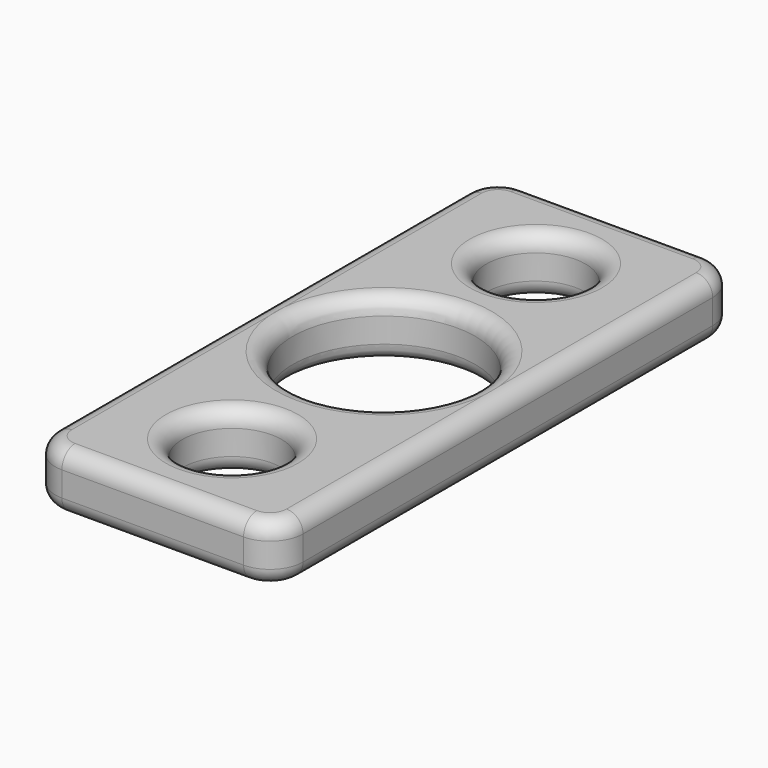
from build123d import *

# Parameters (mm, degrees)
F0_W         = 30
F0_H         = 70
F0_R         = 5.9998479486
F0_R_2       = 11.05
F1_DEPTH     = 7
F2_T1_DEPTH  = 80
F2_T3_DEPTH  = 40
F3_T1_DEPTH  = 6.9999999998
F3_T4_ANGLE  = 90
F3_T6_ANGLE  = 90
F3_T8_ANGLE  = 90
F3_T10_ANGLE = 90
F3_T12_ANGLE = 90
F3_T14_ANGLE = 90
F3_T16_ANGLE = 90
F3_T18_ANGLE = 90


# Not quite as in the source:
# - a fillet or chamfer that OpenCascade refuses, or shapes differently, is made with other operations: its cross-section is extruded or revolved along the edge and cut away or added


with BuildPart() as f1:
    # F0 (on Top) → F1 (new body)
    with BuildSketch(Plane.XY):
        Rectangle(F0_W, F0_H)
        with Locations((0, -23)):
            Circle(F0_R, mode=Mode.SUBTRACT)
        Circle(F0_R_2, mode=Mode.SUBTRACT)
        with Locations((0, 23)):
            Circle(F0_R, mode=Mode.SUBTRACT)
    extrude(amount=F1_DEPTH)

    # F2: fillet of radius 2 on 14 edges, made by hand

    # F2_s2 → F2_t1 (cut)
    with BuildSketch(Plane.XZ.offset(-40)):
        with BuildLine():
            ThreePointArc((15, 5), (14.4142135624, 6.4142135624), (13, 7))
            Line((13, 7), (15, 7))
            Line((15, 7), (15, 5))
        make_face()
        with BuildLine():
            ThreePointArc((-15, 5), (-14.4142135624, 6.4142135624), (-13, 7))
            Line((-13, 7), (-15, 7))
            Line((-15, 7), (-15, 5))
        make_face()
        with BuildLine():
            ThreePointArc((15, 2), (14.4142135624, 0.5857864376), (13, 0))
            Line((13, 0), (15, 0))
            Line((15, 0), (15, 2))
        make_face()
        with BuildLine():
            ThreePointArc((-15, 2), (-14.4142135624, 0.5857864376), (-13, 0))
            Line((-13, 0), (-15, 0))
            Line((-15, 0), (-15, 2))
        make_face()
    extrude(amount=F2_T1_DEPTH, mode=Mode.SUBTRACT)

    # F2_s4 → F2_t3 (cut)
    with BuildSketch(Plane.YZ.offset(-20)):
        with BuildLine():
            ThreePointArc((35, 5), (34.4142135624, 6.4142135624), (33, 7))
            Line((33, 7), (35, 7))
            Line((35, 7), (35, 5))
        make_face()
        with BuildLine():
            ThreePointArc((-35, 5), (-34.4142135624, 6.4142135624), (-33, 7))
            Line((-33, 7), (-35, 7))
            Line((-35, 7), (-35, 5))
        make_face()
        with BuildLine():
            ThreePointArc((35, 2), (34.4142135624, 0.5857864376), (33, 0))
            Line((33, 0), (35, 0))
            Line((35, 0), (35, 2))
        make_face()
        with BuildLine():
            ThreePointArc((-35, 2), (-34.4142135624, 0.5857864376), (-33, 0))
            Line((-33, 0), (-35, 0))
            Line((-35, 0), (-35, 2))
        make_face()
    extrude(amount=F2_T3_DEPTH, mode=Mode.SUBTRACT)

    # F2_s5 → F2_t6 (revolve, cut)
    with BuildSketch(Plane.XZ.offset(23)):
        with BuildLine():
            ThreePointArc((5.9998479486, 5), (6.5856343863, 6.4142135624), (7.9998479486, 7))
            Line((7.9998479486, 7), (5.9998479486, 7))
            Line((5.9998479486, 7), (5.9998479486, 5))
        make_face()
    revolve(axis=Axis((0, -23, 7), (0, 0, 1)), mode=Mode.SUBTRACT)

    # F2_s7 → F2_t8 (revolve, cut)
    with BuildSketch(Plane.XZ):
        with BuildLine():
            ThreePointArc((11.05, 5), (11.6357864376, 6.4142135624), (13.05, 7))
            Line((13.05, 7), (11.05, 7))
            Line((11.05, 7), (11.05, 5))
        make_face()
    revolve(axis=Axis((0, 0, 7), (0, 0, 1)), mode=Mode.SUBTRACT)

    # F2_s9 → F2_t10 (revolve, cut)
    with BuildSketch(Plane.XZ.offset(-23)):
        with BuildLine():
            ThreePointArc((5.9998479486, 5), (6.5856343863, 6.4142135624), (7.9998479486, 7))
            Line((7.9998479486, 7), (5.9998479486, 7))
            Line((5.9998479486, 7), (5.9998479486, 5))
        make_face()
    revolve(axis=Axis((0, 23, 7), (0, 0, 1)), mode=Mode.SUBTRACT)

    # F2_s11 → F2_t12 (revolve, cut)
    with BuildSketch(Plane.XZ.offset(23)):
        with BuildLine():
            ThreePointArc((5.9998479486, 2), (6.5856343863, 0.5857864376), (7.9998479486, 0))
            Line((7.9998479486, 0), (5.9998479486, 0))
            Line((5.9998479486, 0), (5.9998479486, 2))
        make_face()
    revolve(axis=Axis((0, -23, 0), (0, 0, 1)), mode=Mode.SUBTRACT)

    # F2_s13 → F2_t14 (revolve, cut)
    with BuildSketch(Plane.XZ):
        with BuildLine():
            ThreePointArc((11.05, 2), (11.6357864376, 0.5857864376), (13.05, 0))
            Line((13.05, 0), (11.05, 0))
            Line((11.05, 0), (11.05, 2))
        make_face()
    revolve(axis=Axis((0, 0, 0), (0, 0, 1)), mode=Mode.SUBTRACT)

    # F2_s15 → F2_t16 (revolve, cut)
    with BuildSketch(Plane.XZ.offset(-23)):
        with BuildLine():
            ThreePointArc((5.9998479486, 2), (6.5856343863, 0.5857864376), (7.9998479486, 0))
            Line((7.9998479486, 0), (5.9998479486, 0))
            Line((5.9998479486, 0), (5.9998479486, 2))
        make_face()
    revolve(axis=Axis((0, 23, 0), (0, 0, 1)), mode=Mode.SUBTRACT)

    # F3: fillet of radius 4 on 4 edges, made by hand

    # F3_s2 → F3_t1 (cut)
    with BuildSketch(Plane.XY):
        with BuildLine():
            ThreePointArc((-11, -35), (-13.8284271247, -33.8284271247), (-15, -31))
            Line((-15, -31), (-15, -35))
            Line((-15, -35), (-11, -35))
        make_face()
        with BuildLine():
            ThreePointArc((15, -31), (13.8284271247, -33.8284271247), (11, -35))
            Line((11, -35), (15, -35))
            Line((15, -35), (15, -31))
        make_face()
        with BuildLine():
            ThreePointArc((15, 31), (13.8284271247, 33.8284271247), (11, 35))
            Line((11, 35), (15, 35))
            Line((15, 35), (15, 31))
        make_face()
        with BuildLine():
            ThreePointArc((-11, 35), (-13.8284271247, 33.8284271247), (-15, 31))
            Line((-15, 31), (-15, 35))
            Line((-15, 35), (-11, 35))
        make_face()
    extrude(amount=F3_T1_DEPTH, mode=Mode.SUBTRACT)

    # F3_s3 → F3_t4 (revolve, cut)
    with BuildSketch(Plane.XZ.offset(-31)):
        with BuildLine():
            ThreePointArc((-13.0000000001, 0), (-14.4142135624, 0.5857864376), (-15, 1.9999999999))
            Line((-15, 1.9999999999), (-15, 0))
            Line((-15, 0), (-13.0000000001, 0))
        make_face()
    revolve(axis=Axis((-11, 31, 0), (0, 0, -1)), revolution_arc=F3_T4_ANGLE, mode=Mode.SUBTRACT)

    # F3_s5 → F3_t6 (revolve, cut)
    with BuildSketch(Plane.YZ.offset(-11)):
        with BuildLine():
            ThreePointArc((33.0000000001, 7), (34.4142135624, 6.4142135624), (35, 5.0000000001))
            Line((35, 5.0000000001), (35, 7))
            Line((35, 7), (33.0000000001, 7))
        make_face()
    revolve(axis=Axis((-11, 31, 7), (0, 0, 1)), revolution_arc=F3_T6_ANGLE, mode=Mode.SUBTRACT)

    # F3_s7 → F3_t8 (revolve, cut)
    with BuildSketch(Plane.YZ.offset(11)):
        with BuildLine():
            ThreePointArc((33.0000000001, 0), (34.4142135624, 0.5857864376), (35, 1.9999999999))
            Line((35, 1.9999999999), (35, 0))
            Line((35, 0), (33.0000000001, 0))
        make_face()
    revolve(axis=Axis((11, 31, 0), (0, 0, -1)), revolution_arc=F3_T8_ANGLE, mode=Mode.SUBTRACT)

    # F3_s9 → F3_t10 (revolve, cut)
    with BuildSketch(Plane.XZ.offset(-31)):
        with BuildLine():
            ThreePointArc((13.0000000001, 7), (14.4142135624, 6.4142135624), (15, 5.0000000001))
            Line((15, 5.0000000001), (15, 7))
            Line((15, 7), (13.0000000001, 7))
        make_face()
    revolve(axis=Axis((11, 31, 7), (0, 0, 1)), revolution_arc=F3_T10_ANGLE, mode=Mode.SUBTRACT)

    # F3_s11 → F3_t12 (revolve, cut)
    with BuildSketch(Plane.XZ.offset(31)):
        with BuildLine():
            ThreePointArc((13.0000000001, 0), (14.4142135624, 0.5857864376), (15, 1.9999999999))
            Line((15, 1.9999999999), (15, 0))
            Line((15, 0), (13.0000000001, 0))
        make_face()
    revolve(axis=Axis((11, -31, 0), (0, 0, -1)), revolution_arc=F3_T12_ANGLE, mode=Mode.SUBTRACT)

    # F3_s13 → F3_t14 (revolve, cut)
    with BuildSketch(Plane.YZ.offset(11)):
        with BuildLine():
            ThreePointArc((-33.0000000001, 7), (-34.4142135624, 6.4142135624), (-35, 5.0000000001))
            Line((-35, 5.0000000001), (-35, 7))
            Line((-35, 7), (-33.0000000001, 7))
        make_face()
    revolve(axis=Axis((11, -31, 7), (0, 0, 1)), revolution_arc=F3_T14_ANGLE, mode=Mode.SUBTRACT)

    # F3_s15 → F3_t16 (revolve, cut)
    with BuildSketch(Plane.YZ.offset(-11)):
        with BuildLine():
            ThreePointArc((-33.0000000001, 0), (-34.4142135624, 0.5857864376), (-35, 1.9999999999))
            Line((-35, 1.9999999999), (-35, 0))
            Line((-35, 0), (-33.0000000001, 0))
        make_face()
    revolve(axis=Axis((-11, -31, 0), (0, 0, -1)), revolution_arc=F3_T16_ANGLE, mode=Mode.SUBTRACT)

    # F3_s17 → F3_t18 (revolve, cut)
    with BuildSketch(Plane.XZ.offset(31)):
        with BuildLine():
            ThreePointArc((-13.0000000001, 7), (-14.4142135624, 6.4142135624), (-15, 5.0000000001))
            Line((-15, 5.0000000001), (-15, 7))
            Line((-15, 7), (-13.0000000001, 7))
        make_face()
    revolve(axis=Axis((-11, -31, 7), (0, 0, 1)), revolution_arc=F3_T18_ANGLE, mode=Mode.SUBTRACT)


solid = f1.part
